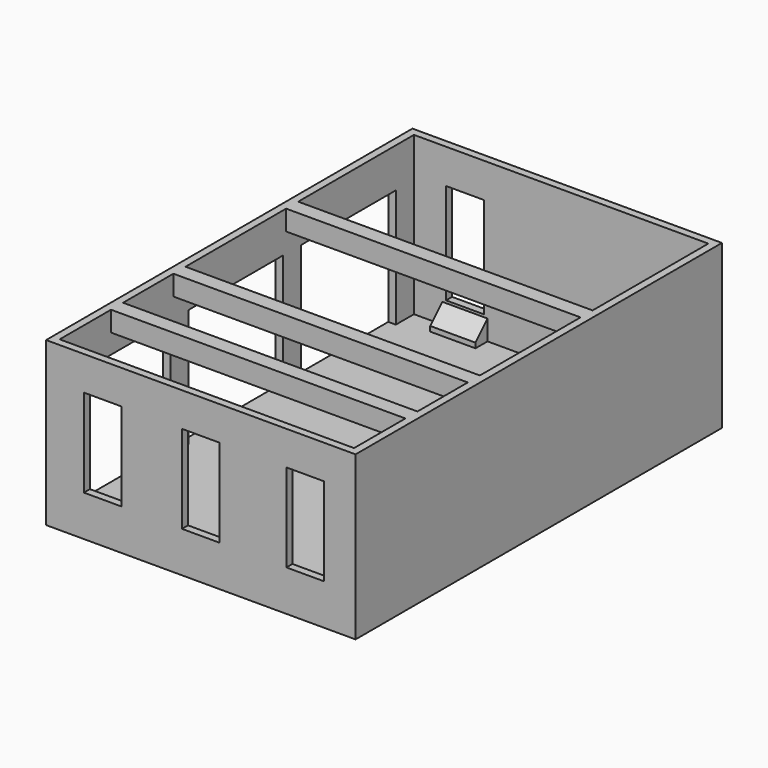
from build123d import *

# Parameters (mm, degrees)
F0_W          = 6248.4
F0_H          = 9245.6
F1_DEPTH      = 3340.1
F1_DEPTH_BACK = 101.6
F3_T          = -152.4
F2_W          = 9245.6
F2_H          = 3441.7
F2_W_2        = 2387.6
F2_H_2        = 2387.6
F4_DEPTH      = 152.4
F5_DEPTH      = 50.8
F6_W          = 914.4
F6_H          = 304.8
F7_DEPTH      = 406.4
F8_SIZE       = 304.79999
F9_W          = 5943.6
F9_H          = 304.8
F10_DEPTH     = 406.4
F11_W         = 762
F11_H         = 1778
F12_DEPTH     = 152.401
F13_W         = 609.6
F13_H         = 508
F14_DEPTH     = 889
F15_W         = 762
F15_H         = 2032
F16_DEPTH     = 152.401
F17_DEPTH     = 152.4


# Not quite as in the source:
# - a fillet or chamfer is up to 0.001 mm smaller than in the source, because OpenCascade refuses the exact size


with BuildPart() as f1:
    # F0 (on Top) → F1 (new body, two sides)
    with BuildSketch(Plane.XY) as f1_sk:
        Rectangle(F0_W, F0_H)
    extrude(amount=F1_DEPTH)
    extrude(f1_sk.sketch, amount=-F1_DEPTH_BACK)

    # F3
    f3_openings = [f1.faces().sort_by_distance(p)[0] for p in [
        (-3124.2, 0, 1619.25),
    ]]
    offset(amount=F3_T, openings=f3_openings)

    # F2 (on face) → F4 (join)
    with BuildSketch(Plane(origin=(-3124.2, 0, 0), x_dir=(0, -1, 0), z_dir=(-1, 0, 0))):
        with Locations((0, 1619.25)):
            Rectangle(F2_W, F2_H)
        with Locations((-2819.4, 1193.8)):
            Rectangle(F2_W_2, F2_H_2, mode=Mode.SUBTRACT)
        with Locations((25.4, 1193.8)):
            Rectangle(F2_W_2, F2_H_2, mode=Mode.SUBTRACT)
        with Locations((2870.2, 1193.8)):
            Rectangle(F2_W_2, F2_H_2, mode=Mode.SUBTRACT)
    extrude(amount=-F4_DEPTH)

    # F5 (cut): a face of the model
    f5_faces = [f1.faces().sort_by_distance(p)[0] for p in [
        (-61.3516059957, -0.5112633833, 50.8),
    ]]
    extrude(f5_faces, amount=-F5_DEPTH, mode=Mode.SUBTRACT)

    # F6 (on face) → F7 (join)
    with BuildSketch(Plane.XY):
        with Locations((-1943.1, 4318)):
            Rectangle(F6_W, F6_H)
    extrude(amount=F7_DEPTH)

    # F8 (size 304.8 in the source; OpenCascade refuses exactly that, so slightly less here)
    f8_edges = [f1.edges().sort_by_distance(p)[0] for p in [
        (-1943.1, 4165.6, 406.4),
    ]]
    chamfer(f8_edges, length=F8_SIZE)

    # F9 (on face) → F10 (join)
    with BuildSketch(Plane(origin=(0, 0, 3187.7), x_dir=(1, 0, 0), z_dir=(0, 0, -1))):
        with Locations((0, 1447.8)):
            Rectangle(F9_W, F9_H)
        with Locations((0, -1397)):
            Rectangle(F9_W, F9_H)
        with Locations((0, 3022.6)):
            Rectangle(F9_W, F9_H)
    extrude(amount=F10_DEPTH)

    # F11 (on face) → F12 (cut, through all)
    with BuildSketch(Plane(origin=(0, -4470.4, 0), x_dir=(-1, 0, 0), z_dir=(0, 1, 0))):
        with Locations((1981.2, 1612.9)):
            Rectangle(F11_W, F11_H)
        with Locations((0, 1612.9)):
            Rectangle(F11_W, F11_H)
        with Locations((-2108.2, 1612.9)):
            Rectangle(F11_W, F11_H)
    extrude(amount=-F12_DEPTH, mode=Mode.SUBTRACT)

    # F13 (on face) → F14 (join)
    with BuildSketch(Plane.XY):
        with Locations((2667, 3962.4)):
            Rectangle(F13_W, F13_H)
    extrude(amount=F14_DEPTH)

    # F15 (on face) → F16 (cut, through all)
    with BuildSketch(Plane.XZ.offset(-4470.4)):
        with Locations((-1943.1, 1473.2)):
            Rectangle(F15_W, F15_H)
    extrude(amount=-F16_DEPTH, mode=Mode.SUBTRACT)

    # F17 (cut): a face of the model
    f17_faces = [f1.faces().sort_by_distance(p)[0] for p in [
        (0, 0, 3340.1),
    ]]
    extrude(f17_faces, amount=-F17_DEPTH, mode=Mode.SUBTRACT)


solid = f1.part
